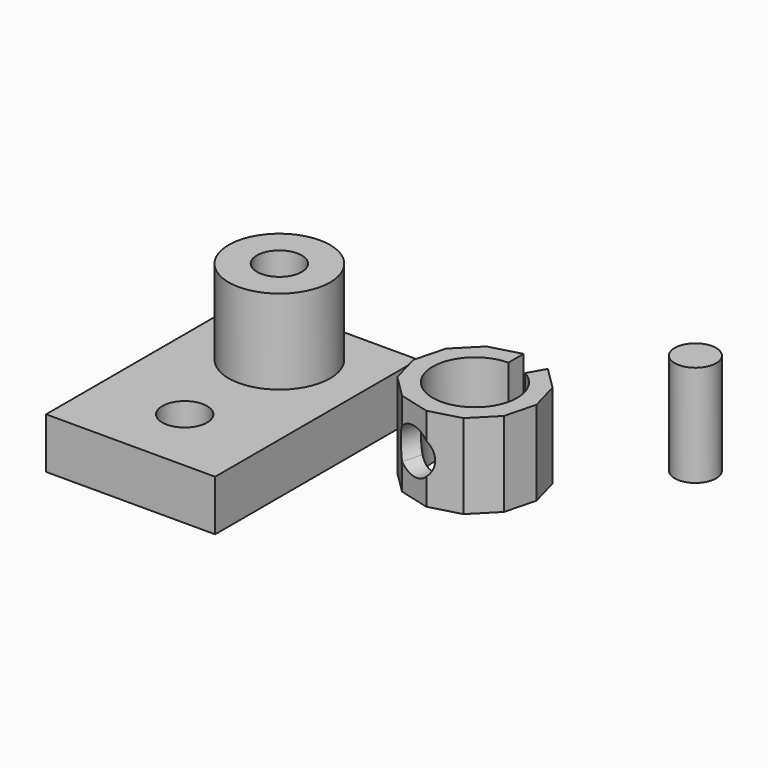
from build123d import *

# Parameters (mm, degrees)
F0_W     = 20
F0_H     = 30
F0_R     = 2.65
F0_R_2   = 6
F1_DEPTH = 6
F2_DEPTH = 10
F3_DEPTH = 10
F5_DEPTH = 2.7610118925
F0_R_3   = 2.45
F6_DEPTH = 12


# Not quite as in the source:
# - a feature names something its author has since deleted; it is built from what else it names


with BuildPart() as f1:
    # F0 (on Top) → F1 (new body)
    with BuildSketch(Plane.XY):
        with Locations((0, 7)):
            Rectangle(F0_W, F0_H)
        Circle(F0_R, mode=Mode.SUBTRACT)
        with Locations((0, 14)):
            Circle(F0_R_2, mode=Mode.SUBTRACT)
        with Locations((0, 14)):
            Circle(F0_R_2)
        with Locations((0, 14)):
            Circle(F0_R, mode=Mode.SUBTRACT)
    extrude(amount=-F1_DEPTH)

    # F0 (on Top) → F2 (join)
    with BuildSketch(Plane.XY):
        with Locations((0, 14)):
            Circle(F0_R_2)
        with Locations((0, 14)):
            Circle(F0_R, mode=Mode.SUBTRACT)
    extrude(amount=F2_DEPTH)


with BuildPart() as f3:
    # F0 (on Top) → F3 (new body)
    with BuildSketch(Plane.XY):
        with BuildLine():
            ThreePointArc((31.4085708903, 11.0953978322), (27.6737183454, 1.912242965), (28.8917668759, 11.750729364))
            Line((28.8917668759, 11.750729364), (28.8917668759, 13.9977169424))
            Line((28.8917668759, 13.9977169424), (25.2739680355, 13.0059012255))
            Line((25.2739680355, 13.0059012255), (22.6367701923, 10.3380641986))
            Line((22.6367701923, 10.3380641986), (21.6868083789, 6.7090506386))
            Line((21.6868083789, 6.7090506386), (22.6786240958, 3.0912517981))
            Line((22.6786240958, 3.0912517981), (25.3464611227, 0.454053955))
            Line((25.3464611227, 0.454053955), (28.9754746827, -0.4959078585))
            Line((28.9754746827, -0.4959078585), (32.5932735232, 0.4959078585))
            Line((32.5932735232, 0.4959078585), (35.2304713663, 3.1637448854))
            Line((35.2304713663, 3.1637448854), (36.1804331798, 6.7927584454))
            Line((36.1804331798, 6.7927584454), (35.1886174628, 10.4105572858))
            Line((35.1886174628, 10.4105572858), (32.5207804359, 13.047755129))
            Line((32.5207804359, 13.047755129), (31.4085708903, 11.0953978322))
        make_face()
    extrude(amount=F3_DEPTH)

    # F4 (on face) → F5 (cut, through all)
    with BuildSketch(Plane(origin=(1.7366663624, 6.63435697, 0), x_dir=(0.9674044991, -0.2532361252, 0), z_dir=(-0.2532361252, -0.9674044991, 0))):
        with BuildLine():
            Line((28.1565863562, 6.8720198406), (28.1565863562, 3.1279801594))
            ThreePointArc((28.1565863562, 3.1279801594), (28.7297128763, 3.9870729344), (28.9309420092, 5))
            ThreePointArc((28.9309420092, 5), (28.7297128763, 6.0129270656), (28.1565863562, 6.8720198406))
        make_face()
        with BuildLine():
            Line((24.4052976622, 6.8720198406), (24.4052976622, 3.1279801594))
            ThreePointArc((24.4052976622, 3.1279801594), (26.2809420092, 2.35), (28.1565863562, 3.1279801594))
            Line((28.1565863562, 3.1279801594), (28.1565863562, 6.8720198406))
            ThreePointArc((28.1565863562, 6.8720198406), (26.2809420092, 7.65), (24.4052976622, 6.8720198406))
        make_face()
        with BuildLine():
            ThreePointArc((24.4052976622, 6.8720198406), (23.6309420092, 5), (24.4052976622, 3.1279801594))
            Line((24.4052976622, 3.1279801594), (24.4052976622, 6.8720198406))
        make_face()
    extrude(amount=-F5_DEPTH, mode=Mode.SUBTRACT)


with BuildPart() as f6:
    # F0 (on Top) → F6 (new body)
    with BuildSketch(Plane.XY):
        with Locations((43.8999424085, 20.652592666)):
            Circle(F0_R_3)
    extrude(amount=F6_DEPTH)


solid = Compound([f1.part, f3.part, f6.part])
